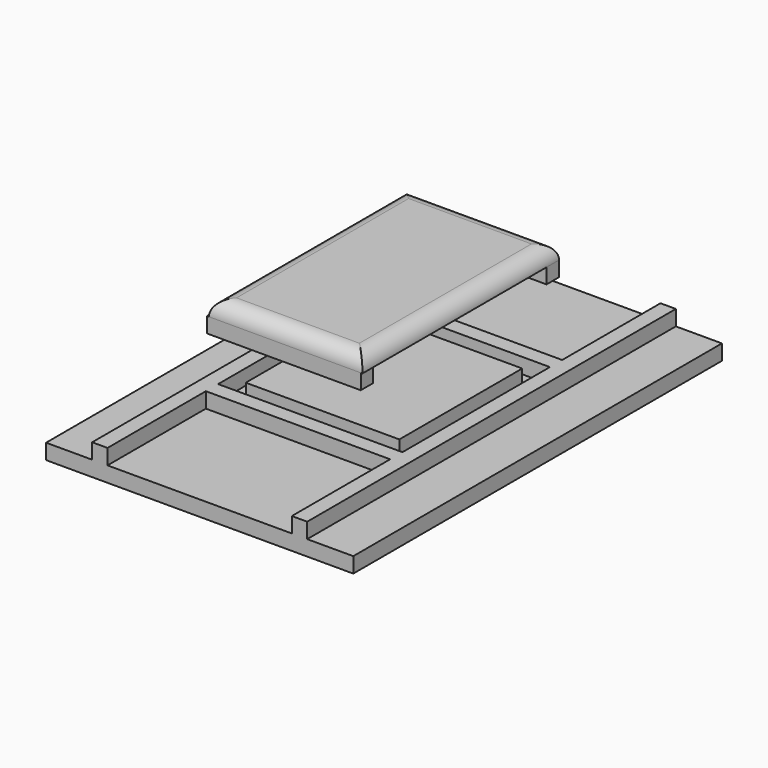
from build123d import *

# Parameters (mm, degrees)
F0_W      = 100
F0_H      = 150
F1_DEPTH  = 5
F3_W      = 60
F3_H      = 5
F4_DEPTH  = 5
F5_W      = 5
F5_H      = 5
F6_DEPTH  = 0.5
F7_W      = 50
F7_H      = 50
F8_DEPTH  = 5
F10_W     = 50
F10_H     = 5
F10_H_2   = 70
F11_DEPTH = 5
F13_W     = 50
F13_H     = 5
F14_DEPTH = 5
F15_R     = 4.99999


# Not quite as in the source:
# - a fillet or chamfer is up to 0.001 mm smaller than in the source, because OpenCascade refuses the exact size


with BuildPart() as f1:
    # F0 (on Top) → F1 (new body)
    with BuildSketch(Plane.XY):
        with Locations((50, 75)):
            Rectangle(F0_W, F0_H)
    extrude(amount=F1_DEPTH)

    # F3 (on offset) → F4 (join)
    with BuildSketch(Plane.XY.offset(5)):
        Polygon((20, 150), (15, 150), (15, 0), (20, 0), (20, 40), (20, 45), (20, 105), (20, 110), align=None)
        with Locations((50, 107.5)):
            Rectangle(F3_W, F3_H)
        Polygon((80, 150), (80, 110), (80, 105), (80, 45), (80, 40), (80, 0), (85, 0), (85, 150), align=None)
        with Locations((50, 42.5)):
            Rectangle(F3_W, F3_H)
    extrude(amount=F4_DEPTH)

    # F5 (on offset) → F6 (cut)
    with BuildSketch(Plane.XY.offset(5)):
        with Locations((22.5, 102.5)):
            Rectangle(F5_W, F5_H)
        with Locations((77.5, 102.5)):
            Rectangle(F5_W, F5_H)
        with Locations((77.5, 47.5)):
            Rectangle(F5_W, F5_H)
        with Locations((22.5, 47.5)):
            Rectangle(F5_W, F5_H)
    extrude(amount=-F6_DEPTH, mode=Mode.SUBTRACT)

    # F7 (on offset) → F8 (join)
    with BuildSketch(Plane.XY.offset(5)):
        with Locations((50, 75)):
            Rectangle(F7_W, F7_H)
    extrude(amount=F8_DEPTH)


with BuildPart() as f11:
    # F10 (on offset) → F11 (new body)
    with BuildSketch(Plane.XY.offset(35)):
        with Locations((50, 112.5)):
            Rectangle(F10_W, F10_H)
        with Locations((50, 75)):
            Rectangle(F10_W, F10_H_2)
        with Locations((50, 37.5)):
            Rectangle(F10_W, F10_H)
    extrude(amount=F11_DEPTH)

    # F13 (on offset) → F14 (join)
    with BuildSketch(Plane(origin=(0, 0, 35), x_dir=(1, 0, 0), z_dir=(0, 0, -1))):
        with Locations((49.4327385849, -37.5)):
            Rectangle(F13_W, F13_H)
        with Locations((49.9044367713, -112.5)):
            Rectangle(F13_W, F13_H)
    extrude(amount=F14_DEPTH)

    # F15 (radius 5 in the source; OpenCascade refuses exactly that, so slightly less here)
    f15_edges = [f11.edges().sort_by_distance(p)[0] for p in [
        (50, 115, 40),
        (25, 75, 40),
        (50, 35, 40),
        (75, 75, 40),
    ]]
    fillet(f15_edges, radius=F15_R)


solid = Compound([f1.part, f11.part])
